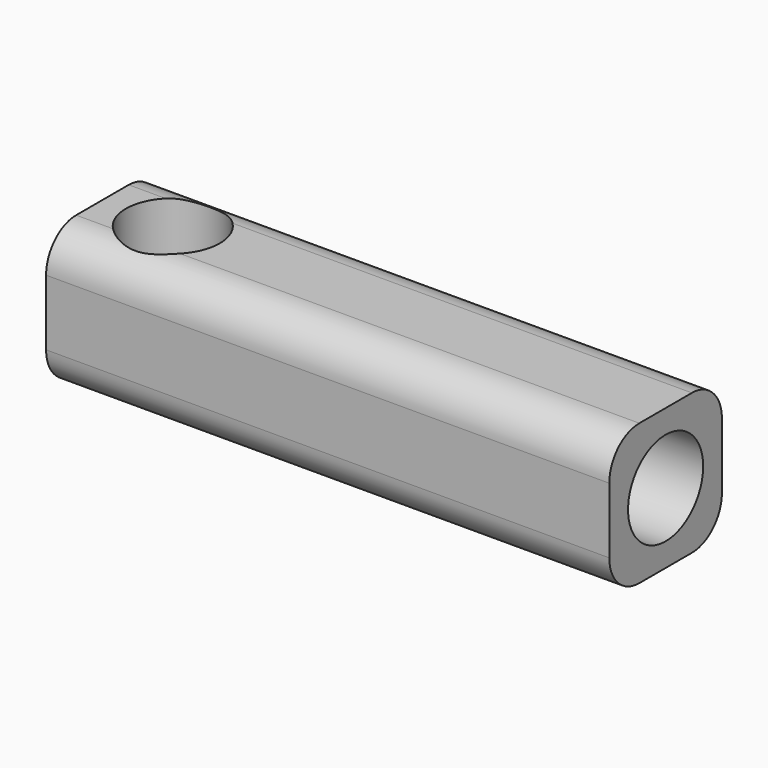
from build123d import *

# Parameters (mm, degrees)
F0_W        = 76.2
F0_H        = 19.05
F1_DEPTH    = 19.05
F3_D        = 12.7
F3_DEPTH    = 39.1412730195
F5_D        = 12.7
F6_T1_DEPTH = 101.6


# Not quite as in the source:
# - a fillet or chamfer that OpenCascade refuses, or shapes differently, is made with other operations: its cross-section is extruded or revolved along the edge and cut away or added


with BuildPart() as f1:
    # F0 (on Top) → F1 (new body)
    with BuildSketch(Plane.XY):
        with Locations((1.0402730195, 0)):
            Rectangle(F0_W, F0_H)
    extrude(amount=F1_DEPTH)

    # F3 (through all, one way)
    with BuildSketch(Plane(origin=(0, 0, 0), x_dir=(0, 1, 0), z_dir=(-1, 0, 0))):
        with Locations((0, -9.525)):
            Circle(F3_D / 2)
    extrude(amount=-F3_DEPTH, mode=Mode.SUBTRACT)

    # F5 (through all)
    with Locations(Plane(origin=(0, 0, 0), x_dir=(1, 0, 0), z_dir=(0, 0, -1))):
        with Locations((-27.5347269805, 0)):
            Hole(F5_D / 2)

    # F6: fillet of radius 5.08 on 4 edges, made by hand

    # F6_s2 → F6_t1 (cut)
    with BuildSketch(Plane.YZ.offset(-49.7597269805)):
        with BuildLine():
            ThreePointArc((4.445, 19.05), (8.0371024484, 17.5621024484), (9.525, 13.97))
            Line((9.525, 13.97), (9.525, 19.05))
            Line((9.525, 19.05), (4.445, 19.05))
        make_face()
        with BuildLine():
            ThreePointArc((-9.525, 13.97), (-8.0371024484, 17.5621024484), (-4.445, 19.05))
            Line((-4.445, 19.05), (-9.525, 19.05))
            Line((-9.525, 19.05), (-9.525, 13.97))
        make_face()
        with BuildLine():
            ThreePointArc((-9.525, 5.08), (-8.0371024484, 1.4878975516), (-4.445, 0))
            Line((-4.445, 0), (-9.525, 0))
            Line((-9.525, 0), (-9.525, 5.08))
        make_face()
        with BuildLine():
            ThreePointArc((4.445, 0), (8.0371024484, 1.4878975516), (9.525, 5.08))
            Line((9.525, 5.08), (9.525, 0))
            Line((9.525, 0), (4.445, 0))
        make_face()
    extrude(amount=F6_T1_DEPTH, mode=Mode.SUBTRACT)


solid = f1.part
